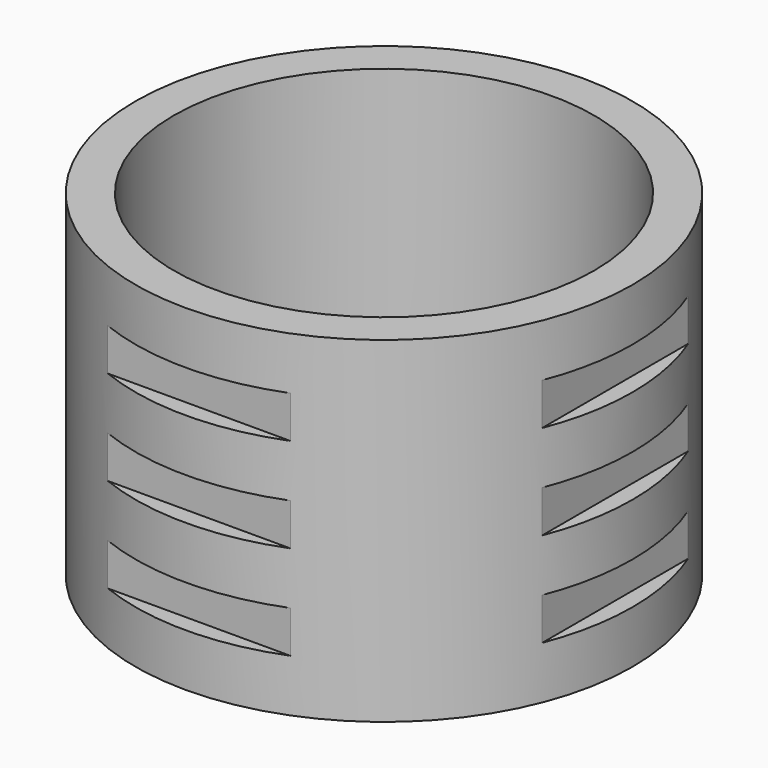
from build123d import *

# Parameters (mm, degrees)
F0_R            = 15.0205390909
F0_R_2          = 12.7
F1_DEPTH        = 20.32
F3_W            = 7.62
F3_H            = 2.54
F4_DEPTH        = 25.4
F4_DEPTH_BACK   = 25.4
F4_COPIES_COUNT = 4


# Not quite as in the source:
# - a pattern or mirror of a feature is missing from the dataset's text; its kind, count and spacing are read off the source's solid


with BuildPart() as f1:
    # F0 (on Top) → F1 (new body)
    with BuildSketch(Plane.XY):
        Circle(F0_R)
        Circle(F0_R_2, mode=Mode.SUBTRACT)
    extrude(amount=F1_DEPTH)

    # F3 (on face) → F4 (cut, two sides)
    with BuildSketch(Plane(origin=(0, 0, 0), x_dir=(0, -1, 0), z_dir=(-1, 0, 0))) as f4_sk:
        with Locations((17.78, 10.16)):
            Rectangle(F3_W, F3_H)
        with Locations((17.78, 15.875)):
            Rectangle(F3_W, F3_H)
        with Locations((17.78, 4.445)):
            Rectangle(F3_W, F3_H)
    f4 = extrude(amount=-F4_DEPTH, mode=Mode.SUBTRACT) + extrude(f4_sk.sketch, amount=F4_DEPTH_BACK, mode=Mode.SUBTRACT)

    # F4_copies: F4 ×4 about axis
    f4_copies_axis = Axis((0, 0, 0), (0, 0, 1))
    for i in range(1, F4_COPIES_COUNT):
        add(f4.rotate(f4_copies_axis, i * 360 / F4_COPIES_COUNT), mode=Mode.SUBTRACT)


solid = f1.part
